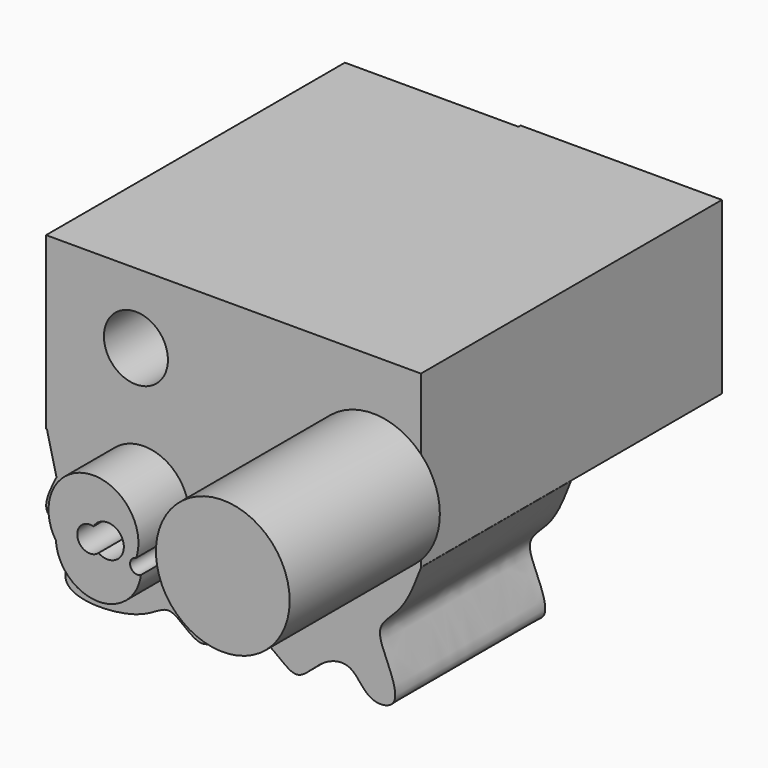
from build123d import *

# Parameters (mm, degrees)
F0_W     = 69.8219751939
F0_H     = 150.2394899726
F1_DEPTH = 68.59726
F2_R     = 12.8812272084
F3_DEPTH = 151.3262167573
F4_R     = 26.8964003772
F5_DEPTH = 75.50996
F7_DEPTH = 75.3914266825
F9_DEPTH = 25.4


with BuildPart() as f1:
    # F0 (on Top) → F1 (new body)
    with BuildSketch(Plane.XY):
        with Locations((-40.0729221292, -0.2716816962)):
            Rectangle(F0_W, F0_H)
        Polygon((-5.1619345322, 75.9347900748), (-5.1619345322, 74.8480632901), (-5.1619345322, -75.3914266825), (75.7989510894, -75.3914266825), (75.7989510894, 75.9347900748), align=None)
    extrude(amount=F1_DEPTH)

    # F2 (on face) → F3 (cut, through all)
    with BuildSketch(Plane.XZ.offset(75.3914266825)):
        with Locations((-38.8503558934, 40.3446033597)):
            Circle(F2_R)
    extrude(amount=-F3_DEPTH, mode=Mode.SUBTRACT)

    # F4 (on face) → F5 (join)
    with BuildSketch(Plane.XZ.offset(75.3914266825)):
        with Locations((56.5096065402, 21.326944232)):
            Circle(F4_R)
    extrude(amount=F5_DEPTH)

    # F6 (on Front) → F7 (join, through all)
    with BuildSketch(Plane.XZ):
        with BuildLine():
            Line((75.8700966835, 0), (-74.64107126, 0))
            add(Edge.make_bspline(
                [(-74.64107126, 0), (-72.9126029737, -7.3674764553), (-70.9594494157, -15.6926583323), (-70.6173188851, -15.7833341551), (-80.6738152373, -32.8577218178), (-58.0686003133, -31.1053232814), (-76.9174521915, -58.2615700065), (-34.8797382228, -56.3076878967), (-25.3744876623, -43.9321196667), (-12.3150093194, -60.9295650154), (-0.7495613738, -45.9497959156), (14.7541074853, -44.777992492), (25.7337633251, -58.7998809192), (35.2733321455, -45.3527476777), (48.6408816788, -42.2778519684), (53.9424871458, -55.0023934283), (68.5151278913, -53.2194204495), (62.2900101587, -37.4864836461), (56.8683509523, -26.0822931742), (69.0009897861, -17.945361749), (73.4010867544, -6.4502237339), (75.8700966835, 0)],
                knots=[0, 0, 0, 0, 0.0588608355, 0.0665122127, 0.1206156222, 0.1700113783, 0.2304494763, 0.3104144422, 0.3641902712, 0.4188897172, 0.4751033368, 0.5304624864, 0.5839550906, 0.6366520196, 0.6859979285, 0.7358494378, 0.7800533718, 0.8345897942, 0.8842954302, 0.9350751281, 1, 1, 1, 1], degree=3))
        make_face()
    extrude(amount=F7_DEPTH)

    # F8 (on face) → F9 (join)
    with BuildSketch(Plane.XZ.offset(75.3914266825)):
        with BuildLine():
            ThreePointArc((-18.4031426907, -16.9800519943), (-38.0179633899, 6.5044832962), (-50.7331602275, -21.326944232))
            ThreePointArc((-50.7331602275, -21.326944232), (-34.109662302, -37.3807196819), (-16.5013764054, -22.4136672914))
            ThreePointArc((-16.5013764054, -22.4136672914), (-20.7064474929, -20.8358259814), (-18.4031426907, -16.9800519943))
        make_face()
        with BuildLine():
            ThreePointArc((-33.5636629552, -20.1817365138), (-41.9913061102, -17.5267023799), (-35.6084015467, -11.4166365264))
            ThreePointArc((-35.6084015467, -11.4166365264), (-23.5532874106, -13.2254475806), (-33.5636629552, -20.1817365138))
        make_face(mode=Mode.SUBTRACT)
    extrude(amount=F9_DEPTH)


solid = f1.part
